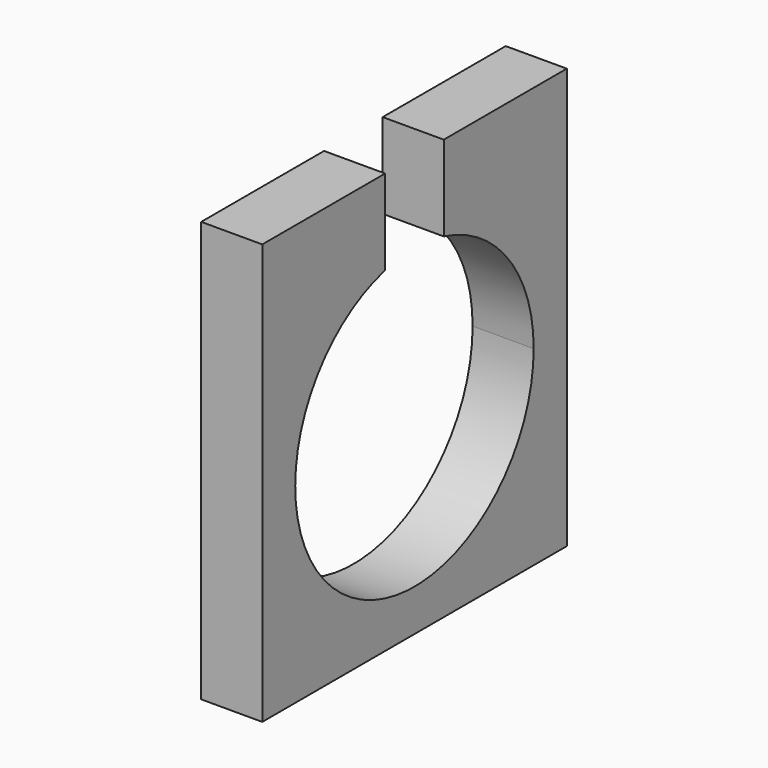
from build123d import *

# Parameters (mm, degrees)
F0_W     = 60.96
F0_H     = 63.5
F1_DEPTH = 6.35
F3_DEPTH = 6.351
F6_DEPTH = 6.351
F7_W     = 39.5752452314
F7_H     = 11.9200152457
F8_DEPTH = 6.351


# Not quite as in the source:
# - a feature of the source that left no trace in its solid (it failed there, or was rolled back) is left out


with BuildPart() as f1:
    # F0 (on Right) → F1 (new body)
    with BuildSketch(Plane.YZ):
        Rectangle(F0_W, F0_H)
    extrude(amount=F1_DEPTH)

    # F2 (on face) → F3 (cut, through all)
    with BuildSketch(Plane.YZ.offset(6.35)):
        with BuildLine():
            ThreePointArc((-3.81, 15.0182534271), (-9.5139869666, -12.2289855671), (15.494, 0))
            ThreePointArc((15.494, 0), (12.2289855671, 9.5139869666), (3.81, 15.0182534271))
            Line((3.81, 15.0182534271), (-3.81, 15.0182534271))
        make_face()
        with BuildLine():
            Line((-3.81, 15.0182534271), (3.81, 15.0182534271))
            ThreePointArc((3.81, 15.0182534271), (0, 15.494), (-3.81, 15.0182534271))
        make_face()
        with BuildLine():
            ThreePointArc((-3.81, 15.0182534271), (0, 15.494), (3.81, 15.0182534271))
            Line((3.81, 15.0182534271), (3.81, 24.1368534271))
            Line((3.81, 24.1368534271), (-3.81, 24.1368534271))
            Line((-3.81, 24.1368534271), (-3.81, 15.0182534271))
        make_face()
    extrude(amount=-F3_DEPTH, mode=Mode.SUBTRACT)

    # F5 (on face) → F6 (cut, through all)
    with BuildSketch(Plane.YZ.offset(6.35)):
        Polygon((30.48, 31.75), (-30.48, 31.75), (-30.48, 23.876), (-3.81, 23.876), (-3.81, 24.1368534271), (3.81, 24.1368534271), (3.81, 23.876), (30.48, 23.876), align=None)
    extrude(amount=-F6_DEPTH, mode=Mode.SUBTRACT)

    # F7 (on face) → F8 (cut, through all)
    with BuildSketch(Plane.YZ.offset(6.35)):
        Polygon((-19.7760853916, 23.876), (-30.48, 23.876), (-30.48, -31.75), (-19.7760853916, -31.75), (-19.7760853916, -19.8299847543), align=None)
        Polygon((19.7991598397, 23.876), (19.7991598397, -19.8299847543), (19.7991598397, -31.75), (30.48, -31.75), (30.48, 23.876), align=None)
        with Locations((0.0115372241, -25.7899923772)):
            Rectangle(F7_W, F7_H)
    extrude(amount=-F8_DEPTH, mode=Mode.SUBTRACT)


solid = f1.part
